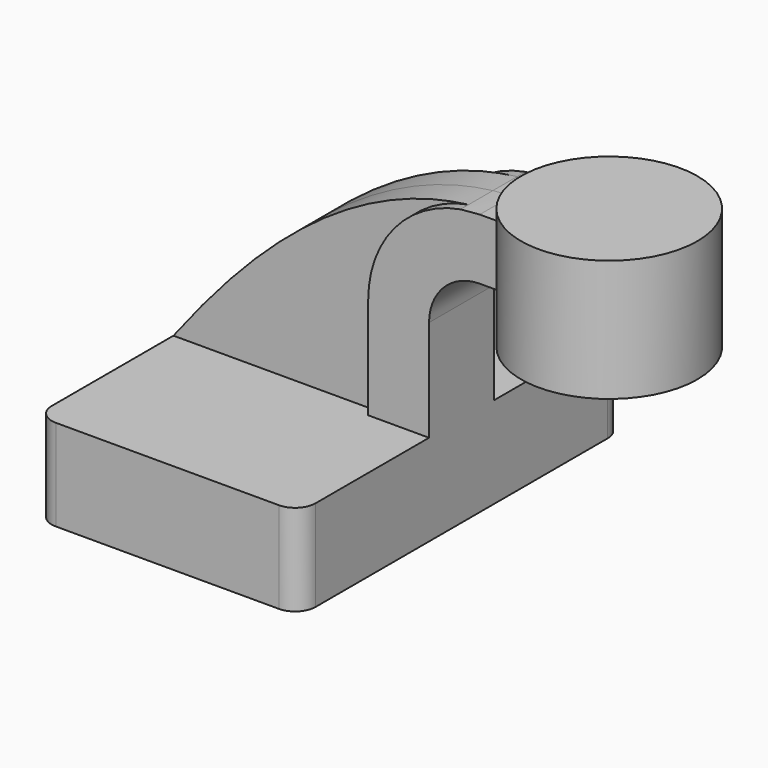
from build123d import *

# Parameters (mm, degrees)
F1_DEPTH = 63.5
F2_DEPTH = 9.525
F0_W     = 27.5973672049
F0_H     = 19.05
F3_DEPTH = 12.7
F5_R     = 6.35


with BuildPart() as f1:
    # F0 (on Front) → F1 (new body, symmetric)
    with BuildSketch(Plane.XZ):
        Polygon((22.225, 14.2875), (-41.275, 14.2875), (-41.275, -14.2875), (41.275, -14.2875), (41.275, 14.2875), align=None)
    extrude(amount=F1_DEPTH, both=True)

    # F0 (on Front) → F2 (join, symmetric)
    with BuildSketch(Plane.XZ):
        with BuildLine():
            add(Edge.make_bspline(
                [(-41.275, 14.2875), (-17.0139536123, 46.0103167382), (13.0965037161, 75.7513709268), (51.1069528866, 80.4357151657)],
                knots=[0, 0, 0, 0, 112.9609338605, 112.9609338605, 112.9609338605, 112.9609338605], degree=3))
            Line((-41.275, 14.2875), (22.225, 14.2875))
            Line((22.225, 14.2875), (22.225, 46.0375))
            ThreePointArc((22.225, 46.0375), (30.4029530094, 68.4952626286), (51.1069528866, 80.4357151657))
        make_face()
    extrude(amount=F2_DEPTH, both=True)

    # F0 (on Front) → F3 (join, symmetric)
    with BuildSketch(Plane.XZ):
        with BuildLine():
            Line((22.225, 46.0375), (22.225, 14.2875))
            Line((22.225, 14.2875), (41.275, 14.2875))
            Line((41.275, 14.2875), (41.275, 46.0375))
            ThreePointArc((41.275, 46.0375), (45.9246798487, 57.2628201513), (57.15, 61.9125))
            Line((57.15, 61.9125), (59.9153243124, 61.9125))
            Line((59.9153243124, 61.9125), (59.9153243124, 80.9625))
            Line((59.9153243124, 80.9625), (57.15, 80.9625))
            add(Edge.make_bspline(
                [(51.1069528866, 80.4357151657), (53.0994946773, 80.6812726864), (55.1137452531, 80.8579756133), (57.15, 80.9625)],
                knots=[112.9609338605, 112.9609338605, 112.9609338605, 112.9609338605, 118.8824471905, 118.8824471905, 118.8824471905, 118.8824471905], degree=3))
            ThreePointArc((51.1069528866, 80.4357151657), (30.4029530094, 68.4952626286), (22.225, 46.0375))
        make_face()
        with Locations((73.7140079149, 71.4375)):
            Rectangle(F0_W, F0_H)
    extrude(amount=F3_DEPTH, both=True)

    # F0 (on Front) → F4 (revolve)
    with BuildSketch(Plane.XZ):
        Polygon((87.5126915174, 87.3125), (87.5126915174, 80.9625), (87.5126915174, 61.9125), (87.5126915174, 49.2125), (115.1100587223, 49.2125), (115.1100587223, 87.3125), align=None)
    revolve(axis=Axis((87.5126915174, 0, 68.2625), (0, 0, 1)))

    # F5
    f5_edges = [f1.edges().sort_by_distance(p)[0] for p in [
        (-41.275, 63.5, 0),
        (41.275, 63.5, 0),
        (41.275, -63.5, 0),
        (-41.275, -63.5, 0),
    ]]
    fillet(f5_edges, radius=F5_R)


solid = f1.part
